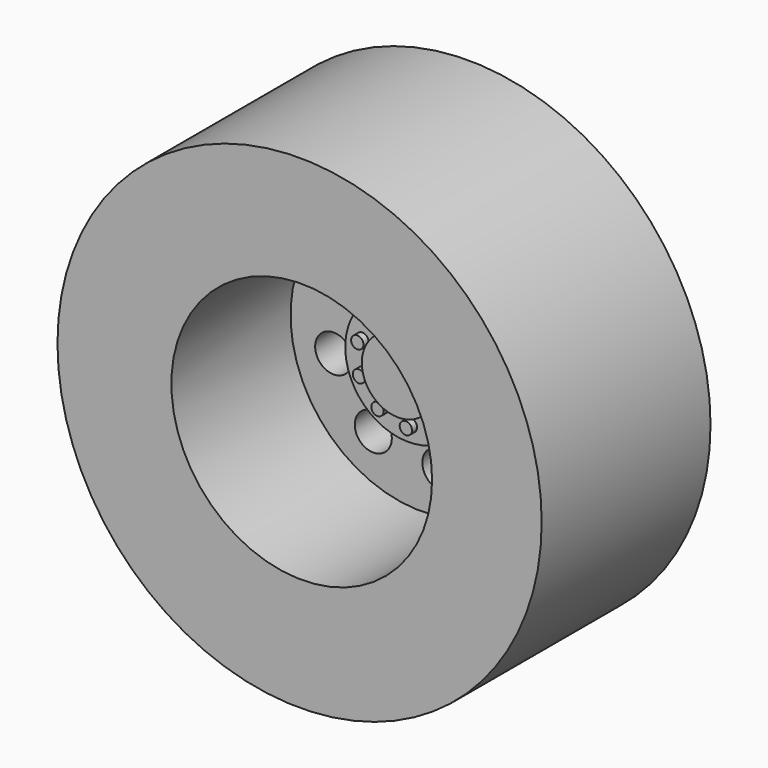
from build123d import *

# Parameters (mm, degrees)
F0_R      = 19.499961
F2_DEPTH  = 16.9999914
F1_R      = 10.5000044
F3_DEPTH  = 12.0000014
F4_R      = 1.4916301958
F5_DEPTH  = 25.4
F7_R      = 17.78
F7_R_2    = 10.7683059636
F8_DEPTH  = 14.9999954
F9_R      = 5.08
F10_DEPTH = 1.27
F13_R     = 2.9336630642
F14_DEPTH = 1.016
F15_R     = 0.4966201378
F16_DEPTH = 0.508


# Not quite as in the source:
# - the program builds the solid bodies; features that only make, move or delete a surface that nothing else refers to are left out


with BuildPart() as f2:
    # F0 (on Front) → F2 (new body)
    with BuildSketch(Plane.XZ):
        with Locations((8.1280004233, 26.7970003188)):
            Circle(F0_R)
    extrude(amount=-F2_DEPTH)

    # F1 (on face) → F3 (cut)
    with BuildSketch(Plane.XZ):
        with Locations((8.3016715726, 26.9168310782)):
            Circle(F1_R)
    extrude(amount=-F3_DEPTH, mode=Mode.SUBTRACT)

    # F4 (on face) → F5 (cut)
    with BuildSketch(Plane.XZ.offset(-12.0000014)):
        with Locations((6.6975592636, 33.9452400804)):
            Circle(F4_R)
        with Locations((12.1372285474, 33.0209454361)):
            Circle(F4_R)
        with Locations((15.3300805747, 28.5209433873)):
            Circle(F4_R)
        with Locations((14.4057859305, 23.0812741034)):
            Circle(F4_R)
        with Locations((9.9057838817, 19.8884220761)):
            Circle(F4_R)
        with Locations((4.4661145978, 20.8127167204)):
            Circle(F4_R)
        with Locations((1.2732625705, 25.3127187692)):
            Circle(F4_R)
        with Locations((2.1975572148, 30.7523880531)):
            Circle(F4_R)
    extrude(amount=-F5_DEPTH, mode=Mode.SUBTRACT)

    # F7 (on face) → F8 (cut)
    with BuildSketch(Plane(origin=(0, 16.9999914, 0), x_dir=(-1, 0, 0), z_dir=(0, 1, 0))):
        with Locations((-8.0529511662, 27.0102884156)):
            Circle(F7_R)
        with Locations((-8.0660926178, 26.997640729)):
            Circle(F7_R_2, mode=Mode.SUBTRACT)
    extrude(amount=-F8_DEPTH, mode=Mode.SUBTRACT)

    # F9 (on face) → F10 (join)
    with BuildSketch(Plane.XZ.offset(-12.0000014)):
        with Locations((8.3016715726, 26.9168310782)):
            Circle(F9_R)
    extrude(amount=F10_DEPTH)

    # F13 (on face) → F14 (join)
    with BuildSketch(Plane.XZ.offset(-10.7300014)):
        with Locations((8.3016715726, 26.9168310782)):
            Circle(F13_R)
    extrude(amount=F14_DEPTH)

    # F15 (on face) → F16 (join)
    with BuildSketch(Plane.XZ.offset(-10.7300014)):
        with Locations((8.092216216, 30.7409893721)):
            Circle(F15_R)
        with Locations((10.3800024772, 30.1337548968)):
            Circle(F15_R)
        with Locations((11.8739369726, 28.297764862)):
            Circle(F15_R)
        with Locations((12.0033875021, 25.934305058)):
            Circle(F15_R)
        with Locations((10.7189083633, 23.9461367989)):
            Circle(F15_R)
        with Locations((8.5111269292, 23.0926727844)):
            Circle(F15_R)
        with Locations((6.2233406681, 23.6999072597)):
            Circle(F15_R)
        with Locations((4.7294061726, 25.5358972945)):
            Circle(F15_R)
        with Locations((4.5999556431, 27.8993570985)):
            Circle(F15_R)
        with Locations((5.884434782, 29.8875253576)):
            Circle(F15_R)
    extrude(amount=F16_DEPTH)


solid = f2.part
